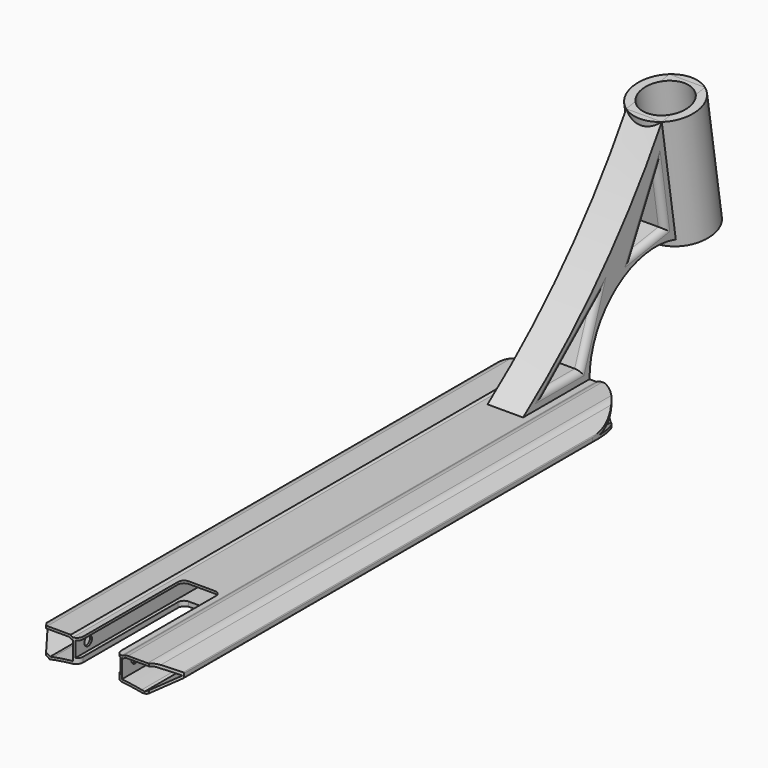
from build123d import *

# Parameters (mm, degrees)
F1_DEPTH       = 250
F2_W           = 38
F2_H           = 13
F3_DEPTH       = 250
F4_T1_DEPTH    = 500
F5_R           = 9
F6_R           = 1
F8_DEPTH       = 500.001
F10_DEPTH      = 526
F10_DEPTH_BACK = 24.001
F12_DEPTH      = 24.0010001
F12_DEPTH_BACK = 527
F13_T1_DEPTH   = 2
F13_T6_DEPTH   = 16.76348167
F13_S7_R       = 200
F13_T8_DEPTH   = 11
F13_T12_DEPTH  = 16.7498753356
F13_S13_R      = 200
F13_T14_DEPTH  = 11
F13_T15_DEPTH  = 26.9727873313
F13_T17_DEPTH  = 27
F15_DEPTH      = 15
F16_R          = 27.5
F17_DEPTH      = 100
F19_D          = 40
F21_D          = 8
F21_DEPTH      = 50
F21_TIP        = 2.4034424761
F23_DEPTH      = 72.5010001
F24_R          = 4.99999


# Not quite as in the source:
# - a fillet or chamfer that OpenCascade refuses, or shapes differently, is made with other operations: its cross-section is extruded or revolved along the edge and cut away or added
# - a fillet or chamfer is up to 0.001 mm smaller than in the source, because OpenCascade refuses the exact size
# - an extrude ends at something that could not be found from the text; its depth is read off the source's solid


with BuildPart() as f1:
    # F0 (on Front) → F1 (new body, symmetric)
    with BuildSketch(Plane.XZ):
        with BuildLine():
            Line((22.5, 22.7), (0, 22.7))
            Line((0, 22.7), (-22.5, 22.7))
            Line((-22.5, 22.7), (-22.5, 24))
            Line((-22.5, 24), (-45.5824640741, 24))
            Line((-45.5824640741, 24), (-57.5, 14))
            Line((-57.5, 14), (-57.5, 10))
            Line((-57.5, 10), (-40.1794919243, 0))
            ThreePointArc((-40.1794919243, 0), (0, 4.0775448584), (40.1794919243, 0))
            Line((40.1794919243, 0), (57.5, 10))
            Line((57.5, 10), (57.5, 14))
            Line((57.5, 14), (45.5824640741, 24))
            Line((45.5824640741, 24), (22.5, 24))
            Line((22.5, 24), (22.5, 22.7))
        make_face()
    extrude(amount=F1_DEPTH, both=True)

    # F2 (on Front) → F3 (cut, symmetric)
    with BuildSketch(Plane.XZ):
        with Locations((0, 14.2)):
            Rectangle(F2_W, F2_H)
    extrude(amount=F3_DEPTH, both=True, mode=Mode.SUBTRACT)

    # F4: fillet of radius 2 on 2 edges, made by hand

    # F4_s2 → F4_t1 (join)
    with BuildSketch(Plane.XZ.offset(-250)):
        with BuildLine():
            ThreePointArc((-20.6265006005, 22.7), (-21.7666760256, 23.0568323275), (-22.5, 24))
            Line((-22.5, 24), (-22.537469988, 23.986))
            ThreePointArc((-22.537469988, 23.986), (-22.54, 23.35), (-22.54, 22.7))
            Line((-22.54, 22.7), (-22.5, 22.66))
            Line((-22.5, 22.66), (-20.6265006005, 22.66))
            Line((-20.6265006005, 22.66), (-20.6265006005, 22.7))
        make_face()
        with BuildLine():
            ThreePointArc((22.5, 24), (21.7666760256, 23.0568323275), (20.6265006005, 22.7))
            Line((20.6265006005, 22.7), (20.6265006005, 22.66))
            Line((20.6265006005, 22.66), (22.5, 22.66))
            Line((22.5, 22.66), (22.54, 22.7))
            ThreePointArc((22.54, 22.7), (22.54, 23.35), (22.537469988, 23.986))
            Line((22.537469988, 23.986), (22.5, 24))
        make_face()
    extrude(amount=F4_T1_DEPTH)

    # F5
    f5_edges = [f1.edges().sort_by_distance(p)[0] for p in [
        (22.5, 0, 24),
        (45.582464, 0, 24),
        (-45.582464, 0, 24),
        (40.179492, 0, 0),
    ]]
    fillet(f5_edges, radius=F5_R)

    # F6
    f6_edges = [f1.edges().sort_by_distance(p)[0] for p in [
        (-57.5, 0, 14),
        (-57.5, 0, 10),
        (57.5, 0, 14),
        (57.5, 0, 10),
    ]]
    fillet(f6_edges, radius=F6_R)

    # F7 (on face) → F8 (cut, through all)
    with BuildSketch(Plane.XZ.offset(250)):
        with BuildLine():
            ThreePointArc((-37.3093701274, 2.6021299876), (-28.9931861118, 3.9860118104), (-20.6265006005, 5.0216850392))
            Line((-20.6265006005, 5.0216850392), (-20.6265006005, 20.7))
            ThreePointArc((-20.6265006005, 20.7), (-22.2389521501, 21.0393989565), (-23.5777715132, 22))
            Line((-23.5777715132, 22), (-42.3067319657, 22))
            ThreePointArc((-42.3067319657, 22), (-44.7008729689, 21.5778483455), (-46.8062452335, 20.3623111018))
            Line((-46.8062452335, 20.3623111018), (-56.850336602, 11.934317739))
            Line((-56.850336602, 11.934317739), (-39.8353828834, 2.1107296294))
            ThreePointArc((-39.8353828834, 2.1107296294), (-38.5731590339, 2.360452347), (-37.3093701274, 2.6021299876))
        make_face()
        with BuildLine():
            ThreePointArc((20.6265006005, 5.0216850392), (28.9931861118, 3.9860118104), (37.3093701274, 2.6021299876))
            ThreePointArc((37.3093701274, 2.6021299876), (38.5731590339, 2.360452347), (39.8353828834, 2.1107296294))
            Line((39.8353828834, 2.1107296294), (56.850336602, 11.934317739))
            Line((56.850336602, 11.934317739), (46.8062452335, 20.3623111018))
            ThreePointArc((46.8062452335, 20.3623111018), (44.7008729689, 21.5778483455), (42.3067319657, 22))
            Line((42.3067319657, 22), (23.5777715132, 22))
            ThreePointArc((23.5777715132, 22), (22.2389521501, 21.0393989565), (20.6265006005, 20.7))
            Line((20.6265006005, 20.7), (20.6265006005, 5.0216850392))
        make_face()
    extrude(amount=-F8_DEPTH, mode=Mode.SUBTRACT)

    # F9 (on Top) → F10 (cut, two sides)
    with BuildSketch(Plane.XY) as f10_sk:
        with BuildLine():
            ThreePointArc((-57.5, 200), (0, 257.5), (57.5, 200))
            Line((57.5, 200), (57.5, 280))
            Line((57.5, 280), (-57.5, 280))
            Line((-57.5, 280), (-57.5, 200))
        make_face()
    extrude(amount=-F10_DEPTH, mode=Mode.SUBTRACT)
    extrude(f10_sk.sketch, amount=F10_DEPTH_BACK, mode=Mode.SUBTRACT)

    # F11 (on Top) → F12 (cut, two sides)
    with BuildSketch(Plane.XY) as f12_sk:
        Polygon((68, -216), (43.2759711825, -250.0297062655), (15.9999905109, -250), (15.9999905109, -140), (-15.9999905109, -139.9651488265), (-16.1197914197, -249.965083589), (-43.3229223053, -249.965083589), (-68, -216), (-68, -345.0383526169), (68, -346), align=None)
    extrude(amount=F12_DEPTH, mode=Mode.SUBTRACT)
    extrude(f12_sk.sketch, amount=-F12_DEPTH_BACK, mode=Mode.SUBTRACT)

    # F13: fillet of radius 5 on 6 edges, made by hand

    # F13_s2 → F13_t1 (join)
    with BuildSketch(Plane.XY.offset(20.7)):
        with BuildLine():
            ThreePointArc((-10.9999934762, -139.9705943224), (-14.5371202342, -141.4312090009), (-16.0054360068, -144.9651458612))
            Line((-16.0054360068, -144.9651458612), (-15.9999905109, -139.9651488265))
            Line((-15.9999905109, -139.9651488265), (-10.9999934762, -139.9705943224))
        make_face()
        with BuildLine():
            ThreePointArc((15.9999905109, -144.9945574663), (14.5374491664, -141.4609493583), (11.0054360068, -139.9945604316))
            Line((11.0054360068, -139.9945604316), (15.9999905109, -140))
            Line((15.9999905109, -140), (15.9999905109, -144.9945574663))
        make_face()
    extrude(amount=F13_T1_DEPTH)


with BuildPart() as f13_tool4:
    # F13_s5 → F13_t6 (new body)
    with BuildSketch(Plane.XY.offset(-9.06348167)):
        with BuildLine():
            ThreePointArc((-16.0054360068, -144.9651458612), (-14.5371202342, -141.4312090009), (-10.9999934762, -139.9705943224))
            Line((-10.9999934762, -139.9705943224), (-15.9999905109, -139.9651488265))
            Line((-15.9999905109, -139.9651488265), (-16.0054360068, -144.9651458612))
        make_face()
    extrude(amount=F13_T6_DEPTH)

    # F13_s7 → F13_t8 (cut, symmetric)
    with BuildSketch(Plane.XZ.offset(142.5)):
        with Locations((0, -195.9224551416)):
            Circle(F13_S7_R)
    extrude(amount=F13_T8_DEPTH, both=True, mode=Mode.SUBTRACT)


with BuildPart() as f1_1:
    add(f1.part)

    # F13_t3: union F13_tool4
    add(f13_tool4.part)


with BuildPart() as f13_tool10:
    # F13_s11 → F13_t12 (new body)
    with BuildSketch(Plane.XY.offset(-9.0498753356)):
        with BuildLine():
            ThreePointArc((15.9999905109, -144.9945574663), (14.5374491664, -141.4609493583), (11.0054360068, -139.9945604316))
            Line((11.0054360068, -139.9945604316), (15.9999905109, -140))
            Line((15.9999905109, -140), (15.9999905109, -144.9945574663))
        make_face()
    extrude(amount=F13_T12_DEPTH)

    # F13_s13 → F13_t14 (cut, symmetric)
    with BuildSketch(Plane.XZ.offset(142.5)):
        with Locations((0, -195.9224551416)):
            Circle(F13_S13_R)
    extrude(amount=F13_T14_DEPTH, both=True, mode=Mode.SUBTRACT)


with BuildPart() as f1_2:
    add(f1_1.part)

    # F13_t9: union F13_tool10
    add(f13_tool10.part)

    # F13_s16 → F13_t15 (cut)
    with BuildSketch(Plane.XY.offset(8.2136063343)):
        with BuildLine():
            ThreePointArc((-21.1143488859, -249.965083589), (-17.580740778, -248.5025422445), (-16.1143518513, -244.9705290848))
            Line((-16.1143518513, -244.9705290848), (-16.1197914197, -249.965083589))
            Line((-16.1197914197, -249.965083589), (-21.1143488859, -249.965083589))
        make_face()
    extrude(amount=F13_T15_DEPTH, mode=Mode.SUBTRACT)

    # F13_s18 → F13_t17 (cut)
    with BuildSketch(Plane.XY.offset(8.2)):
        with BuildLine():
            ThreePointArc((20.9999905109, -250), (17.464456605, -248.5355339059), (15.9999905109, -245))
            Line((15.9999905109, -245), (15.9999905109, -250))
            Line((15.9999905109, -250), (20.9999905109, -250))
        make_face()
    extrude(amount=F13_T17_DEPTH, mode=Mode.SUBTRACT)

    # F14 (on Right) → F15 (join, symmetric)
    with BuildSketch(Plane.YZ):
        with BuildLine():
            ThreePointArc((326.2546872889, 182.7), (261.0880436995, 95.4231893928), (180, 22.7))
            Line((180, 22.7), (250, 22.7))
            ThreePointArc((250, 22.7), (278.5963190182, 79.142317468), (341.0210057474, 89.4691344662))
            Line((341.0210057474, 89.4691344662), (341.8981337929, 83.9311659405))
            Line((341.8981337929, 83.9311659405), (387.3317974603, 91.1271513323))
            Line((387.3317974603, 91.1271513323), (371.6883509563, 189.8959853919))
            Line((371.6883509563, 189.8959853919), (326.2546872889, 182.7))
        make_face()
    extrude(amount=F15_DEPTH, both=True)

    # F16 (on face) → F17 (join)
    with BuildSketch(Plane(origin=(0, -20.2446819507, 127.8198913302), x_dir=(1, 0, 0), z_dir=(0, -0.156434465, 0.9876883406))):
        with Locations((0, 373.8185274626)):
            Circle(F16_R)
    extrude(amount=-F17_DEPTH)

    # F19 (through all)
    with Locations(Plane(origin=(0, -20.2446819507, 127.8198913302), x_dir=(1, 0, 0), z_dir=(0, -0.156434465, 0.9876883406))):
        with Locations((0, 373.8185274626)):
            Hole(F19_D / 2)

    # F21 (one way)
    with BuildSketch(Plane.YZ.offset(20.6265006005)):
        with Locations((-235.9860310154, 15.0216850392)):
            Circle(F21_D / 2)
    extrude(amount=-F21_DEPTH, mode=Mode.SUBTRACT)
    with Locations(Plane.YZ.offset(20.6265006005)):
        with Locations((-235.9860310154, 15.0216850392)):
            with Locations((0, 0, -(F21_DEPTH + F21_TIP / 2))):  # 118° drill point
                Cone(0, F21_D / 2, F21_TIP, mode=Mode.SUBTRACT)

    # F22 (on face) → F23 (cut, through all)
    with BuildSketch(Plane.YZ.offset(15)):
        Polygon((321.8047505779, 146.558919862), (296.2505862651, 96.9506071889), (328.8443015047, 102.1129445352), align=None)
        Polygon((206.6274606681, 32.7), (240.6274606681, 32.7), (256.0183671177, 74.9861679354), align=None)
    extrude(amount=-F23_DEPTH, mode=Mode.SUBTRACT)

    # F24 (radius 5 in the source; OpenCascade refuses exactly that, so slightly less here)
    f24_edges = [f1_2.edges().sort_by_distance(p)[0] for p in [
        (15, 231.322914, 53.843084),
        (15, 223.627461, 32.7),
        (15, 248.322914, 53.843084),
        (-15, 248.322914, 53.843084),
        (-15, 231.322914, 53.843084),
        (-15, 223.627461, 32.7),
        (-15, 312.547444, 99.531776),
        (15, 312.547444, 99.531776),
        (-15, 325.324526, 124.335932),
        (-15, 309.027668, 121.754764),
        (15, 309.027668, 121.754764),
        (15, 325.324526, 124.335932),
        (15.999991, -250, 5.568259),
        (-16.119791, -249.965084, 5.563434),
    ]]
    fillet(f24_edges, radius=F24_R)


solid = f1_2.part
